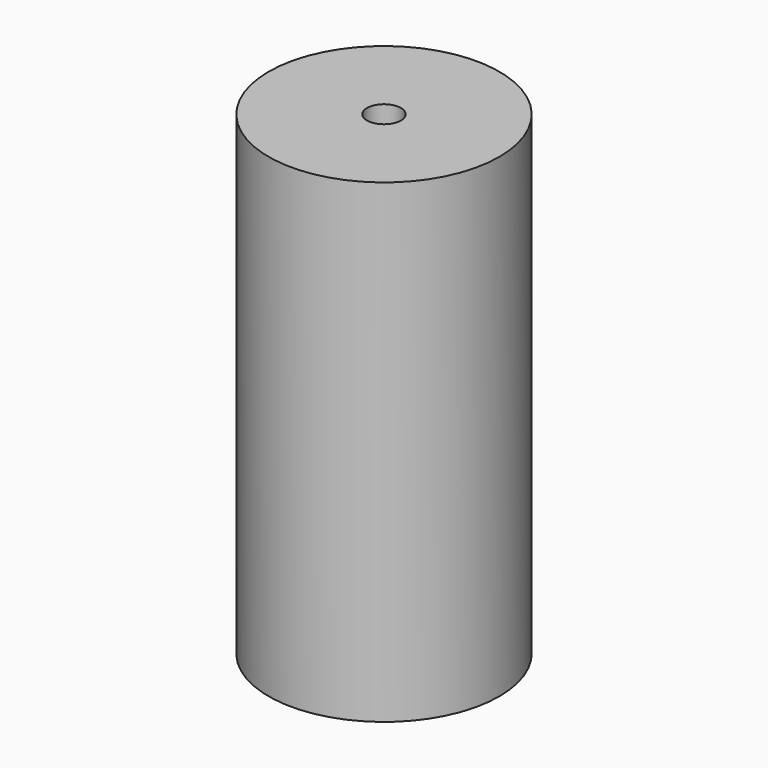
from build123d import *


# Not quite as in the source:
# - a feature names something its author has since deleted; it is built from what else it names


with BuildPart() as f1:
    # F0 (on Front) → F1 (revolve)
    with BuildSketch(Plane.XZ):
        with BuildLine():
            Line((-15, 25.5), (-13, 25.5))
            Line((-13, 25.5), (-2.5, 25.5))
            Line((-2.5, 25.5), (-2.5, 28.5))
            Line((-2.5, 28.5), (-17, 28.5))
            Line((-17, 28.5), (-17, -41.5))
            Line((-17, -41.5), (0, -41.5))
            Line((0, -41.5), (0, -38.5))
            ThreePointArc((0, -38.5), (-9.1923881554, -34.6923881554), (-13, -25.5))
            Line((-13, -25.5), (-13, 22.5))
            Line((-13, 22.5), (-15, 22.5))
            Line((-15, 22.5), (-15, 25.5))
        make_face()
    revolve(axis=Axis((0, 0, -33.5), (0, 0, 1)))


solid = f1.part
